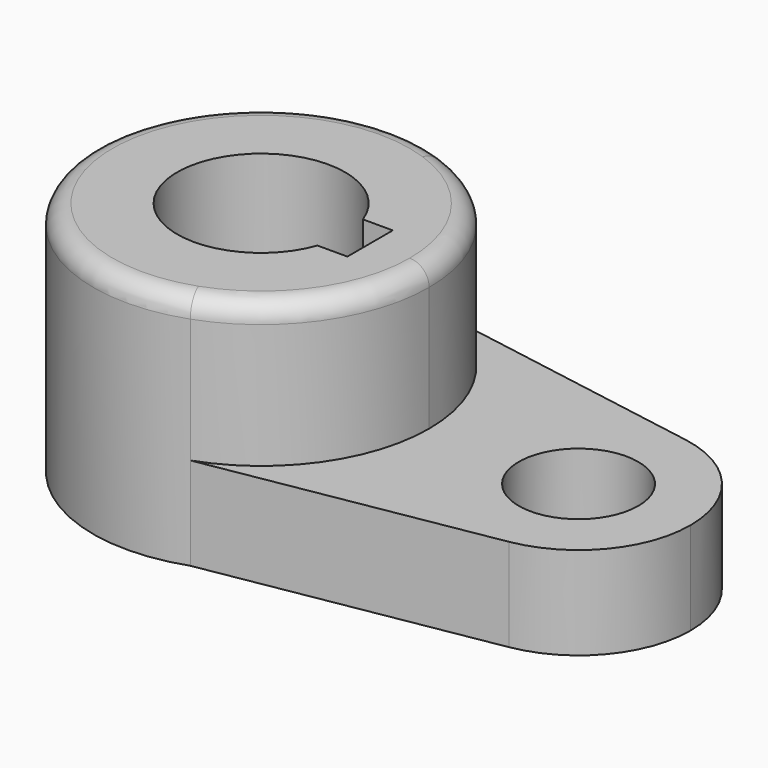
from build123d import *

# Parameters (mm, degrees)
F1_DEPTH = 40.2336
F0_R     = 10.16
F2_DEPTH = 15.7734
F3_R     = 3.302


with BuildPart() as f1:
    # F0 (on Top) → F1 (new body)
    with BuildSketch(Plane.XY):
        with BuildLine():
            ThreePointArc((-19.1519816242, -26.9452959039), (-5.3367005723, -16.5033322905), (-0.0891661078, 0))
            ThreePointArc((-0.0891661078, 0), (-5.3367005723, 16.5033322905), (-19.1519816242, 26.9452959039))
            ThreePointArc((-19.1519816242, 26.9452959039), (-57.2391661078, 0), (-19.1519816242, -26.9452959039))
        make_face()
        with BuildLine():
            ThreePointArc((-15.2164012284, -4.826), (-42.9516661078, 0), (-15.2164012284, 4.826))
            Line((-15.2164012284, 4.826), (-10.1348661078, 4.826))
            Line((-10.1348661078, 4.826), (-10.1348661078, -4.826))
            Line((-10.1348661078, -4.826), (-15.2164012284, -4.826))
        make_face(mode=Mode.SUBTRACT)
    extrude(amount=F1_DEPTH)

    # F0 (on Top) → F2 (join)
    with BuildSketch(Plane.XY):
        with BuildLine():
            ThreePointArc((-19.1519816242, 26.9452959039), (-5.3367005723, 16.5033322905), (-0.0891661078, 0))
            ThreePointArc((-0.0891661078, 0), (-5.3367005723, -16.5033322905), (-19.1519816242, -26.9452959039))
            Line((-19.1519816242, -26.9452959039), (28.5277611544, -18.7764181619))
            ThreePointArc((28.5277611544, -18.7764181619), (6.2608338922, 0), (28.5277611544, 18.7764181619))
            Line((28.5277611544, 18.7764181619), (-19.1519816242, 26.9452959039))
        make_face()
        with BuildLine():
            ThreePointArc((44.3608338922, 0), (39.8742291753, 12.2804730295), (28.5277611544, 18.7764181619))
            ThreePointArc((28.5277611544, 18.7764181619), (6.2608338922, 0), (28.5277611544, -18.7764181619))
            ThreePointArc((28.5277611544, -18.7764181619), (39.8742291753, -12.2804730295), (44.3608338922, 0))
        make_face()
        with Locations((25.3108338922, 0)):
            Circle(F0_R, mode=Mode.SUBTRACT)
    extrude(amount=F2_DEPTH)

    # F3
    f3_edges = [f1.edges().sort_by_distance(p)[0] for p in [
        (-38.176351, 26.945296, 40.2336),
    ]]
    fillet(f3_edges, radius=F3_R)


solid = f1.part
